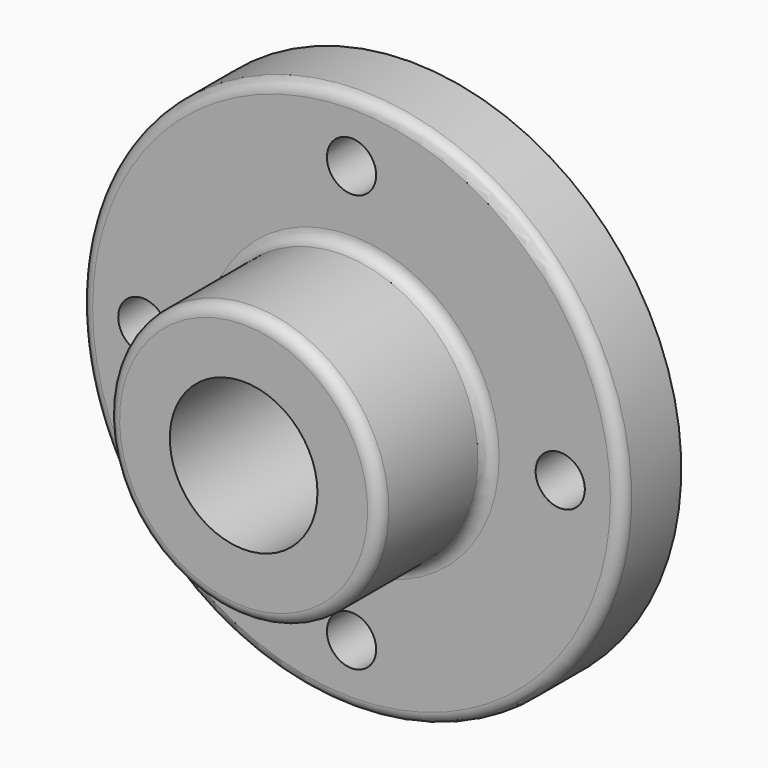
from build123d import *

# Parameters (mm, degrees)
F2_R            = 19.05
F3_DEPTH        = 53.849
F4_R            = 3.048
F5_R            = 6.35
F6_DEPTH        = 19.051
F6_COPIES_COUNT = 4


# Not quite as in the source:
# - a pattern or mirror of a feature is missing from the dataset's text; its kind, count and spacing are read off the source's solid


with BuildPart() as f1:
    # F0 (on Right) → F1 (revolve)
    with BuildSketch(Plane.YZ):
        Polygon((0, 35.052), (0, 0), (53.848, 0), (53.848, 69.85), (34.798, 69.85), (34.798, 35.052), align=None)
    revolve(axis=Axis((0, 38.2506623864, 0), (0, 1, 0)))

    # F2 (on Front) → F3 (cut, through all)
    with BuildSketch(Plane.XZ):
        Circle(F2_R)
    extrude(amount=-F3_DEPTH, mode=Mode.SUBTRACT)

    # F4
    f4_edges = [f1.edges().sort_by_distance(p)[0] for p in [
        (0, 0, -35.052),
        (0, 34.798, -35.052),
        (0, 34.798, -69.85),
    ]]
    fillet(f4_edges, radius=F4_R)

    # F5 (on face) → F6 (cut, through all)
    with BuildSketch(Plane.XZ.offset(-34.798)):
        with Locations((0, 53.848)):
            Circle(F5_R)
    f6 = extrude(amount=-F6_DEPTH, mode=Mode.SUBTRACT)

    # F6_copies: F6 ×4 about axis
    f6_copies_axis = Axis((0, 0, 0), (0, 1, 0))
    for i in range(1, F6_COPIES_COUNT):
        add(f6.rotate(f6_copies_axis, i * 360 / F6_COPIES_COUNT), mode=Mode.SUBTRACT)


solid = f1.part
